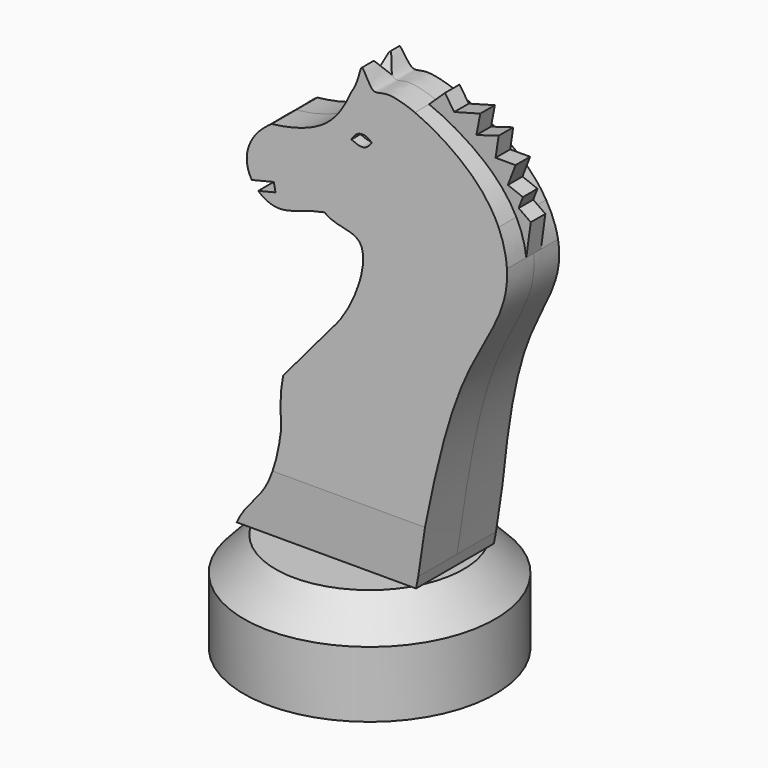
from build123d import *

# Parameters (mm, degrees)
F0_W          = 20.6789579242
F0_H          = 10.8552348391
F2_DEPTH      = 8
F2_DEPTH_BACK = 8
F4_D          = 2
F4_DEPTH      = 0.02
F4_TIP        = 0.600860619
F6_DEPTH      = 5
F8_DEPTH      = 50
F9_DEPTH      = 5
F10_DEPTH     = 1.5


# Not quite as in the source:
# - a feature names something its author has since deleted; it is built from what else it names


with BuildPart() as f1:
    # F0 (on Front) → F1 (revolve)
    with BuildSketch(Plane.XZ):
        with Locations((-10.3394789621, -37.3608471565)):
            Rectangle(F0_W, F0_H)
        Polygon((0, -31.9332297369), (0, -26.4121625388), (-15.4678484998, -26.4121625388), (-20.6789579242, -31.9332297369), align=None)
    revolve(axis=Axis((0, 0, -34.6003135574), (0, 0, -1)))

    # F0 (on Front) → F2 (join, two sides)
    with BuildSketch(Plane.XZ) as f2_sk:
        with BuildLine():
            Line((14.038357413, -26.4121625388), (14.3952110409, -24.5715194245))
            add(Edge.make_bspline(
                [(14.3952110409, -24.5715194245), (15.9619608326, -13.7814918894), (18.8021590043, 5.4666552278), (26.9978979539, 15.993717288), (27.1144497599, 21.8914681421), (26.9814962231, 23.0904583244)],
                knots=[0, 0, 0, 0, 0.1156844152, 0.1975646049, 0.2181556218, 0.2181556218, 0.2181556218, 0.2181556218], degree=3))
            add(Edge.make_bspline(
                [(26.9814962231, 23.0904583244), (26.7846905821, 24.8652740757), (26.2452436001, 26.6704814655), (25.344876099, 28.4262529159)],
                knots=[0.2181556218, 0.2181556218, 0.2181556218, 0.2181556218, 0.2486356554, 0.2486356554, 0.2486356554, 0.2486356554], degree=3))
            add(Edge.make_bspline(
                [(25.344876099, 28.4262529159), (24.5051345796, 30.0638000105), (21.0186712804, 34.8825157579), (14.5296114059, 38.7170585643), (10.98781587, 40.0967356116)],
                knots=[0.2486356554, 0.2486356554, 0.2486356554, 0.2486356554, 0.277063325, 0.3345441119, 0.3345441119, 0.3345441119, 0.3345441119], degree=3))
            add(Edge.make_bspline(
                [(10.98781587, 40.0967356116), (9.163334328, 40.8074472495), (5.7640582422, 41.6424023418), (3.9352599619, 40.0284444481), (1.6363018619, 45.5934628318), (1.8130037382, 41.5469846141), (0.5343510683, 39.659168793)],
                knots=[0.3345441119, 0.3345441119, 0.3345441119, 0.3345441119, 0.3641541314, 0.3969760657, 0.4336110016, 0.4766483866, 0.4766483866, 0.4766483866, 0.4766483866], degree=3))
            add(Edge.make_bspline(
                [(-12.1636614203, 31.1329476535), (-8.2767362316, 31.5887067044), (-2.6053656166, 33.3557904876), (-0.295862871, 37.6032754322), (0.5343510683, 39.659168793)],
                knots=[0, 0, 0, 0, 0.5496493024, 1, 1, 1, 1], degree=3))
            add(Edge.make_bspline(
                [(-12.1636614203, 31.1329476535), (-12.7750103857, 30.7000832732), (-15.9263811745, 28.1746534038), (-16.4342397075, 24.7924460425), (-15.1466824832, 22.6073882083), (-14.9538682628, 22.3364443727)],
                knots=[0.5521533551, 0.5521533551, 0.5521533551, 0.5521533551, 0.5637453002, 0.6182545828, 0.6264560598, 0.6264560598, 0.6264560598, 0.6264560598], degree=3))
            Line((-14.9538682628, 22.3364443727), (-11.3684702665, 23.1903744077))
            Line((-11.3684702665, 23.1903744077), (-11.0409372519, 21.8151607886))
            Line((-11.0409372519, 21.8151607886), (-13.8421699482, 21.1479944832))
            add(Edge.make_bspline(
                [(-13.8421699482, 21.1479944832), (-12.9268650175, 20.3925372869), (-9.52469711, 18.8671743562), (-6.2369346132, 21.0491882768), (-2.9133421604, 21.5721095844)],
                knots=[0.6397771031, 0.6397771031, 0.6397771031, 0.6397771031, 0.6687443358, 0.7277611632, 0.7277611632, 0.7277611632, 0.7277611632], degree=3))
            add(Edge.make_bspline(
                [(-2.9133421604, 21.5721095844), (0.7371625177, 22.1464660094), (9.9413663151, 21.1145809617), (4.0482261588, 12.1754516168), (0.370119941, 7.5280824079)],
                knots=[0.7277611632, 0.7277611632, 0.7277611632, 0.7277611632, 0.792582951, 0.8470977487, 0.8470977487, 0.8470977487, 0.8470977487], degree=3))
            add(Edge.make_bspline(
                [(0.370119941, 7.5280824079), (-0.0320093873, 6.9481805466), (-0.459463289, 6.4123463038), (-0.905206551, 5.9402141272)],
                knots=[0.5460230959, 0.5460230959, 0.5460230959, 0.5460230959, 0.5927503631, 0.5927503631, 0.5927503631, 0.5927503631], degree=3))
            add(Edge.make_bspline(
                [(-0.905206551, 5.9402141272), (-3.331341758, 2.9577861286), (-6.0489482584, -0.1979987283), (-8.5257704402, -3.2600278808)],
                knots=[0.8532288298, 0.8532288298, 0.8532288298, 0.8532288298, 0.8873823849, 0.8873823849, 0.8873823849, 0.8873823849], degree=3))
            add(Edge.make_bspline(
                [(-8.5257704402, -3.2600278808), (-8.8398658261, -5.128027918), (-8.8625409542, -7.5664133699), (-8.4718540311, -10.8553441241)],
                knots=[0.9000780496, 0.9000780496, 0.9000780496, 0.9000780496, 1, 1, 1, 1], degree=3))
            add(Edge.make_bspline(
                [(-8.4718540311, -10.8553441241), (-9.2752194032, -21.6012336314), (-13.1358503435, -21.2265564006), (-15.4678484998, -26.4121625388)],
                knots=[0, 0, 0, 0, 17.0575067871, 17.0575067871, 17.0575067871, 17.0575067871], degree=3))
            Line((-15.4678484998, -26.4121625388), (0, -26.4121625388))
            Line((0, -26.4121625388), (14.038357413, -26.4121625388))
        make_face()
        with BuildLine():
            add(Edge.make_bspline(
                [(-2.9133421604, 21.5721095844), (-1.1822335938, 20.1210338522), (5.7608439074, 21.435257443), (2.9892261487, 11.3050378749), (0.370119941, 7.5280824079)],
                knots=[0, 0, 0, 0, 0.241684002, 0.5460230959, 0.5460230959, 0.5460230959, 0.5460230959], degree=3))
            add(Edge.make_bspline(
                [(-2.9133421604, 21.5721095844), (0.7371625177, 22.1464660094), (9.9413663151, 21.1145809617), (4.0482261588, 12.1754516168), (0.370119941, 7.5280824079)],
                knots=[0.7277611632, 0.7277611632, 0.7277611632, 0.7277611632, 0.792582951, 0.8470977487, 0.8470977487, 0.8470977487, 0.8470977487], degree=3))
        make_face()
    extrude(amount=F2_DEPTH)
    extrude(f2_sk.sketch, amount=-F2_DEPTH_BACK)

    # F4
    with Locations(Plane.XZ.offset(8)):
        with Locations((2.1857838146, 33.2171469927)):
            Hole(F4_D / 2, depth=F4_DEPTH)
            with Locations((0, 0, -(F4_DEPTH + F4_TIP / 2))):  # 118° drill point
                Cone(0, F4_D / 2, F4_TIP, mode=Mode.SUBTRACT)

    # F5 (on face) → F6 (cut)
    with BuildSketch(Plane(origin=(0, 8, 0), x_dir=(-1, 0, 0), z_dir=(0, 1, 0))):
        with BuildLine():
            add(Edge.make_bspline(
                [(-3.8388320245, 33.7408818305), (-2.2842687344, 34.8101302049), (-0.9907989533, 33.7631323009), (-0.967985709, 33.6834328971), (-0.6477286224, 33.3515368402)],
                knots=[0, 0, 0, 0, 0.6653358907, 1, 1, 1, 1], degree=3))
            add(Edge.make_bspline(
                [(-3.8388320245, 33.7408818305), (-3.2120910473, 32.6519496739), (-2.1882613655, 32.3103889823), (-0.6477286224, 33.3515368402)],
                knots=[0, 0, 0, 0, 3.2147675568, 3.2147675568, 3.2147675568, 3.2147675568], degree=3))
        make_face()
    extrude(amount=-F6_DEPTH, mode=Mode.SUBTRACT)

    # F7 (on Right) → F8 (cut, symmetric)
    with BuildSketch(Plane.YZ):
        Polygon((23.508325438, 51.9029956256), (3.1822129985, 48.1615178287), (8.6014410481, -25.5088619888), (28.9033099751, -21.437811648), align=None)
        Polygon((-8.5280006416, -25.5088619888), (-3.9164805785, 48.1615178287), (-18.9101491123, 50.7681109011), (-18.9101491123, -18.7366958708), align=None)
        Polygon((0, 41.3849018514), (2.6577380486, 45.0094938278), (-2.9235549989, 45.0094938278), align=None)
    extrude(amount=F8_DEPTH, both=True, mode=Mode.SUBTRACT)

    # F3 (on face) → F9 (cut)
    with BuildSketch(Plane.XZ.offset(8)):
        with BuildLine():
            add(Edge.make_bspline(
                [(0.8922034758, 33.0823399127), (1.7268573865, 34.751649946), (3.1576943584, 34.6324145794), (4.2308215052, 33.6387753487)],
                knots=[0, 0, 0, 0, 3.3846699604, 3.3846699604, 3.3846699604, 3.3846699604], degree=3))
            add(Edge.make_bspline(
                [(4.2308215052, 33.6387753487), (3.1974392477, 32.247684896), (2.4820207618, 32.4066691101), (0.8922034758, 33.0823399127)],
                knots=[0, 0, 0, 0, 3.3846699604, 3.3846699604, 3.3846699604, 3.3846699604], degree=3))
        make_face()
    extrude(amount=-F9_DEPTH, mode=Mode.SUBTRACT)

    # F0 (on Front) → F10 (join, symmetric)
    with BuildSketch(Plane.XZ):
        with BuildLine():
            add(Edge.make_bspline(
                [(25.344876099, 28.4262529159), (24.5051345796, 30.0638000105), (21.0186712804, 34.8825157579), (14.5296114059, 38.7170585643), (10.98781587, 40.0967356116)],
                knots=[0.2486356554, 0.2486356554, 0.2486356554, 0.2486356554, 0.277063325, 0.3345441119, 0.3345441119, 0.3345441119, 0.3345441119], degree=3))
            Line((25.344876099, 28.4262529159), (25.7208793492, 29.8506842201))
            Line((25.7208793492, 29.8506842201), (26.4216868583, 31.6727800197))
            Line((26.4216868583, 31.6727800197), (23.9487942308, 32.6238945127))
            Line((23.9487942308, 32.6238945127), (25.2106357366, 35.9046757221))
            Line((25.2106357366, 35.9046757221), (21.9298508018, 35.9046757221))
            Line((21.9298508018, 35.9046757221), (22.4260445684, 39.2587259412))
            Line((22.4260445684, 39.2587259412), (18.775254488, 38.1759889424))
            Line((18.775254488, 38.1759889424), (19.4053892046, 41.4844714105))
            Line((19.4053892046, 41.4844714105), (15.1159185916, 40.3211154044))
            Line((15.1159185916, 40.3211154044), (13.6025529355, 42.5973422825))
            Line((13.6025529355, 42.5973422825), (10.98781587, 40.0967356116))
        make_face()
        with BuildLine():
            add(Edge.make_bspline(
                [(26.9814962231, 23.0904583244), (26.7846905821, 24.8652740757), (26.2452436001, 26.6704814655), (25.344876099, 28.4262529159)],
                knots=[0.2181556218, 0.2181556218, 0.2181556218, 0.2181556218, 0.2486356554, 0.2486356554, 0.2486356554, 0.2486356554], degree=3))
            Line((26.9814962231, 23.0904583244), (27.7151837945, 28.4483451396))
            Line((27.7151837945, 28.4483451396), (25.7208793492, 29.8506842201))
            Line((25.7208793492, 29.8506842201), (25.344876099, 28.4262529159))
        make_face()
    extrude(amount=F10_DEPTH, both=True)


solid = f1.part
